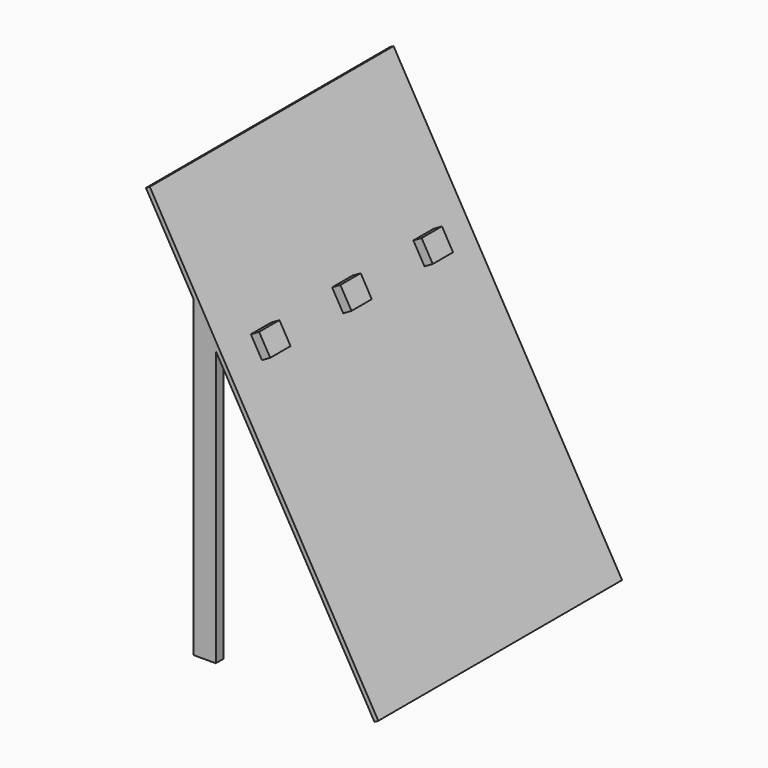
from build123d import *

# Parameters (mm, degrees)
F1_DEPTH = 1219.2
F2_DEPTH = 1219.2
F3_W     = 88.9
F3_H     = 38.1
F6_W     = 101.6
F6_H     = 44.45
F6_W_2   = 50.8
F7_DEPTH = 38.1


# Not quite as in the source:
# - a feature of the source that left no trace in its solid (it failed there, or was rolled back) is left out


with BuildPart() as f1:
    # F0 (on Front) → F1 (new body)
    with BuildSketch(Plane.XZ):
        Polygon((1412.622521745, 0), (1428.0204534243, 8.89), (818.4204534243, 1064.748172294), (803.022521745, 1055.858172294), align=None)
    extrude(amount=F1_DEPTH)

    # F0 (on Front) → F2 (join, through all)
    with BuildSketch(Plane.XZ):
        Polygon((803.022521745, 1055.858172294), (818.4204534243, 1064.748172294), (513.6204534243, 1592.677258441), (498.222521745, 1583.787258441), align=None)
    extrude(amount=F2_DEPTH)

    # F3 (on Top) → F5 (join, up to the next surface of F1)
    with BuildSketch(Plane.XY):
        with Locations((733.172521745, -19.05)):
            Rectangle(F3_W, F3_H)
        with Locations((733.172521745, -1200.15)):
            Rectangle(F3_W, F3_H)
    extrude(until=Until.NEXT)

    # F6 (on face) → F7 (join)
    with BuildSketch(Plane(origin=(1074.864822988, 0, 620.5734948946), x_dir=(0, 1, 0), z_dir=(0.8660254038, 0, 0.5))):
        with Locations((-203.2, 490.6637391275)):
            Rectangle(F6_W, F6_H)
        with Locations((-203.2, 535.1137391275)):
            Rectangle(F6_W, F6_H)
        with Locations((-1016, 490.6637391275)):
            Rectangle(F6_W, F6_H)
        with Locations((-1016, 535.1137391275)):
            Rectangle(F6_W, F6_H)
        Polygon((-558.8, 468.4387391275), (-558.8, 512.8887391275), (-609.6, 512.8887391275), (-660.4, 512.8887391275), (-660.4, 468.4387391275), align=None)
        with Locations((-584.2, 535.1137391275)):
            Rectangle(F6_W_2, F6_H)
        with Locations((-635, 535.1137391275)):
            Rectangle(F6_W_2, F6_H)
    extrude(amount=F7_DEPTH)


solid = f1.part
